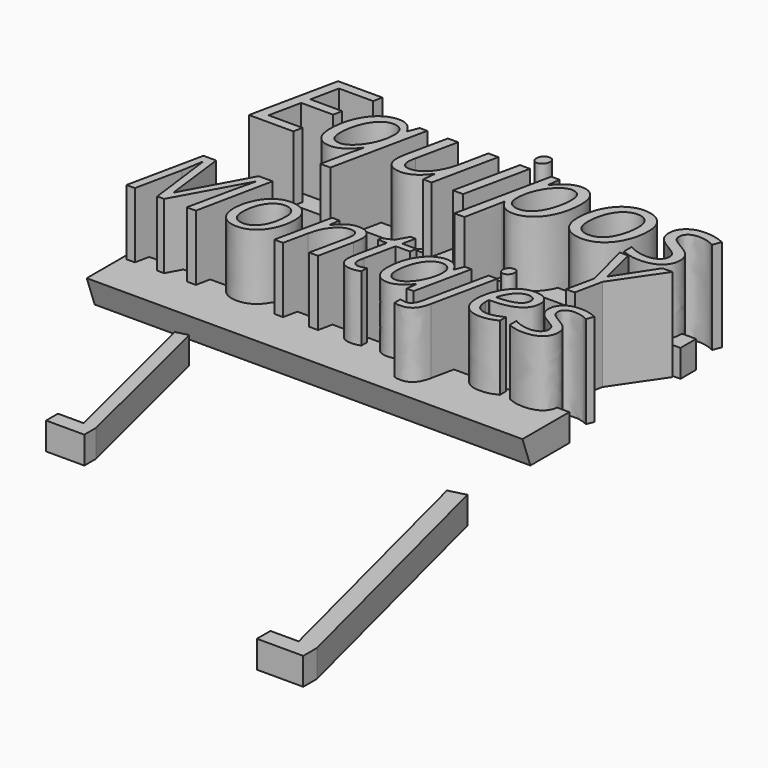
from build123d import *

# Parameters (mm, degrees)
F1_W           = 70.4656625167
F1_H           = 3.5836622119
F1_W_2         = 2.0467182621
F1_W_3         = 7.5528025627
F1_H_2         = 25.4991650581
F1_H_3         = 2.4809986353
F2_DEPTH       = 5
F3_SIZE2       = 1.819841
F3_SIZE        = 4.99999
F0_TEXT_SIZE   = 22.6568722896
F0_TEXT_SIZE_2 = 19.2145184171
F0_TEXT_SIZE_3 = 19.5860908152
F4_DEPTH       = 17
F5_W           = 0.5513317883
F5_H           = 3.514751792
F6_DEPTH       = 8
F5_W_2         = 0.8269995451
F5_H_2         = 3.5147480667
F8_DEPTH       = 5
F10_DEPTH      = 5


# Not quite as in the source:
# - a fillet or chamfer is up to 0.001 mm smaller than in the source, because OpenCascade refuses the exact size
# - Text() gives the source's letters only with a copy of the font that has no kerning and outlines rounded to 1/6400 em; it was checked with that copy


with BuildPart() as f2:
    # F1 (on Top) → F2 (new body)
    with BuildSketch(Plane.XY):
        with Locations((-44.8323520832, 42.6534228027)):
            Rectangle(F1_W, F1_H)
        with Locations((-8.5761616938, 42.6534228027)):
            Rectangle(F1_W_2, F1_H)
        with Locations((-3.7764012814, 42.6534228027)):
            Rectangle(F1_W_3, F1_H)
        with Locations((-8.5761616938, 28.1120091677)):
            Rectangle(F1_W_2, F1_H_2)
        with Locations((-8.5761616938, 14.121927321)):
            Rectangle(F1_W_2, F1_H_3)
        Polygon((-9.5995208248, 12.8814280033), (-9.5995208248, 15.3624266386), (-79.9677148461, 15.3624266386), (-79.9677148461, 4.6114251018), (0, 4.6114251018), (0, 15.3624266386), (-7.5528025627, 15.3624266386), (-7.5528025627, 12.8814280033), align=None)
    extrude(amount=F2_DEPTH)

    # F3 (size 5 and 1.8198511713 in the source; OpenCascade refuses exactly that, so slightly less here)
    f3_edges = [f2.edges().sort_by_distance(p)[0] for p in [
        (-39.983857, 4.611425, 0),
    ]]
    f3_side = f2.faces().sort_by_distance((-39.983857, 4.611425, 2.5))[0]
    chamfer(f3_edges, length=F3_SIZE, length2=F3_SIZE2, reference=f3_side)

    # F0 (on Top) → F4 (join)
    with BuildSketch(Plane.XY):
        with Locations((-80, 40.6816671139)):
            Text('Equipos', F0_TEXT_SIZE, font='Open Sans', font_style=FontStyle.ITALIC, text_align=(TextAlign.LEFT, TextAlign.BOTTOM))
        with Locations((-12.6815821553, 26.8472138536)):
            Text('Y', F0_TEXT_SIZE_2, font='Open Sans', font_style=FontStyle.ITALIC, text_align=(TextAlign.LEFT, TextAlign.BOTTOM))
        with Locations((-80, 12.7452284667)):
            Text('Montajes', F0_TEXT_SIZE_3, font='Open Sans', font_style=FontStyle.ITALIC, text_align=(TextAlign.LEFT, TextAlign.BOTTOM))
    extrude(amount=F4_DEPTH)


with BuildPart() as f6:
    # F5 (on Top) → F6 (new body)
    with BuildSketch(Plane.XY):
        with Locations((-37.6644935459, 53.7532232702)):
            Rectangle(F5_W, F5_H)
    extrude(amount=F6_DEPTH)


with BuildPart() as f6b:
    # F5 (on Top) → F6, piece 2 (new body)
    with BuildSketch(Plane.XY):
        with Locations((-20.090745762, 23.9812266082)):
            Rectangle(F5_W_2, F5_H_2)
    extrude(amount=F6_DEPTH)


with BuildPart() as f8:
    # F7 (on Top) → F8 (new body)
    with BuildSketch(Plane.XY):
        Polygon((-52.1930071599, -30.7982694358), (-56.9168739021, -30.7982694358), (-56.9168739021, -33.5272289813), (-49.8995482922, -33.5272289813), (-49.8995482922, -30.7982694358), align=None)
        Polygon((-59.6634034271, -0.5335962743), (-52.1930071599, -30.7982694358), (-49.8995482922, -30.7982694358), (-57.501655072, 0), align=None)
    extrude(amount=F8_DEPTH)


with BuildPart() as f10:
    # F9 (on Top) → F10 (new body)
    with BuildSketch(Plane.XY):
        Polygon((14.168551811, -64.4318237901), (8.9842099696, -64.4318237901), (8.9842099696, -67.5444677472), (17.4921117723, -67.5444677472), (17.4921117723, -64.4318237901), align=None)
        Polygon((1.5045158067, -14.5926987991), (14.168551811, -64.4318237901), (17.4921117723, -64.4318237901), (4.6265018173, -13.7994075194), align=None)
    extrude(amount=F10_DEPTH)


solid = Compound([f2.part, f6.part, f6b.part, f8.part, f10.part])
